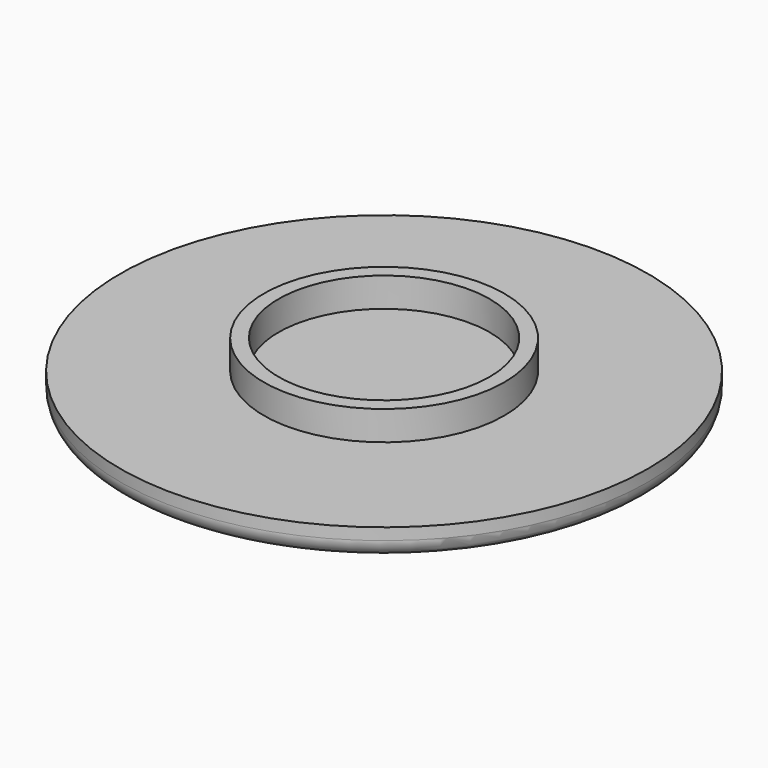
from build123d import *

# Parameters (mm, degrees)
F0_R     = 9
F0_R_2   = 4.1
F1_DEPTH = 1
F0_R_3   = 3.6
F2_DEPTH = 2
F3_R     = 0.6


with BuildPart() as f1:
    # F0 (on Top) → F1 (new body)
    with BuildSketch(Plane.XY):
        Circle(F0_R)
        Circle(F0_R_2, mode=Mode.SUBTRACT)
    extrude(amount=F1_DEPTH)

    # F0 (on Top) → F2 (join)
    with BuildSketch(Plane.XY):
        Circle(F0_R_2)
        Circle(F0_R_3, mode=Mode.SUBTRACT)
    extrude(amount=F2_DEPTH)

    # F3
    f3_edges = [f1.edges().sort_by_distance(p)[0] for p in [
        (-9, 0, 0),
    ]]
    fillet(f3_edges, radius=F3_R)


with BuildPart() as f1b:
    # F0 (on Top) → F1, piece 2 (new body)
    with BuildSketch(Plane.XY):
        Circle(F0_R_3)
    extrude(amount=F1_DEPTH)


solid = Compound([f1.part, f1b.part])
